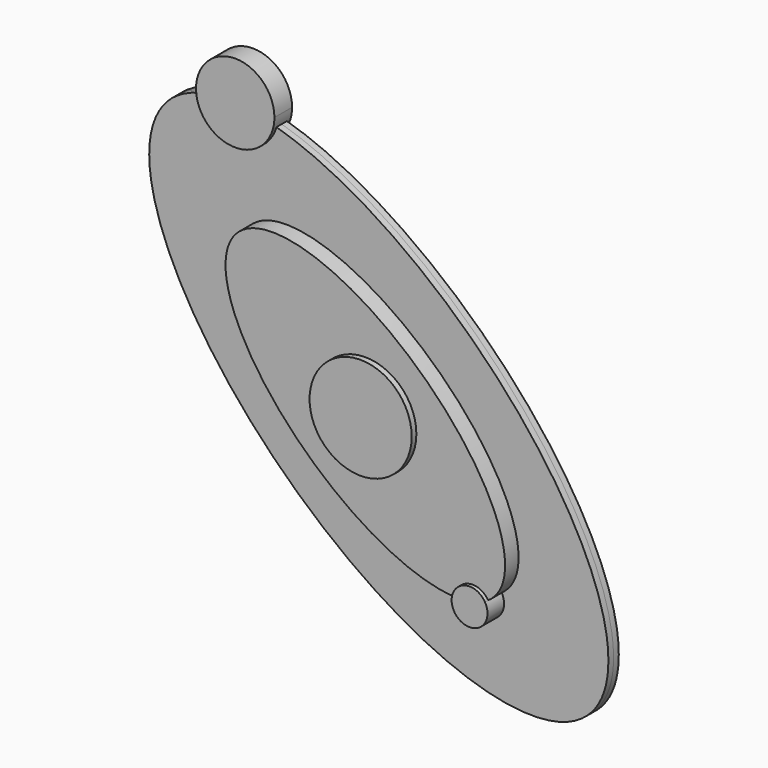
from build123d import *

# Parameters (mm, degrees)
F0_R     = 9.9911429725
F1_DEPTH = 4.572
F2_DEPTH = 1.27
F3_DEPTH = 2.159
F4_DEPTH = 5.334
F5_DEPTH = 5.715


with BuildPart() as f1:
    # F0 (on Front) → F1 (new body, symmetric)
    with BuildSketch(Plane.XZ):
        with BuildLine():
            add(Edge.make_bspline(
                [(24.0256715913, -24.0862835764), (37.8362153163, -14.8498020052), (11.6992033111, 10.0651317638), (-14.4378086941, 34.9800655329), (-25.3313519061, 22.9629725218)],
                knots=[3.0299304445, 3.0299304445, 3.0299304445, 4.6565578758, 4.6565578758, 6.2831853072, 6.2831853072, 6.2831853072], degree=2, weights=[1, 0.68709457, 1, 0.68709457, 1]))
            add(Edge.make_bspline(
                [(-25.3313519061, 22.9629725218), (-33.3755919456, 14.0890571319), (-16.1354711317, -5.4583110371), (1.1046496822, -25.0056792062), (17.5079205841, -25.6094847422)],
                knots=[0, 0, 0, 1.3259269599, 1.3259269599, 2.6518539199, 2.6518539199, 2.6518539199], degree=2, weights=[1, 0.7881718057, 1, 0.7881718057, 1]))
            ThreePointArc((17.5079205841, -25.6094847422), (20.2082141624, -22.4577219219), (24.0256715913, -24.0862835764))
        make_face()
        Circle(F0_R, mode=Mode.SUBTRACT)
    extrude(amount=F1_DEPTH, both=True)

    # F0 (on Front) → F2 (join, symmetric)
    with BuildSketch(Plane.XZ):
        with BuildLine():
            add(Edge.make_bspline(
                [(-34.973748483, 42.7912469007), (-38.9398495635, 41.8233210223), (-41.3951352239, 39.2327047884)],
                knots=[6.003713608, 6.003713608, 6.003713608, 6.2831853072, 6.2831853072, 6.2831853072], degree=2, weights=[1, 0.990252822, 1]))
            add(Edge.make_bspline(
                [(-41.3951352239, 39.2327047884), (-64.7472102278, 14.5935087972), (-5.026258058, -28.7696901063), (54.6946941118, -72.1328890099), (44.2403631424, -22.9469660632), (33.7860321731, 26.2389568835), (-20.0170077048, 41.7593431913)],
                knots=[0, 0, 0, 1.8577548126, 1.8577548126, 3.7155096253, 3.7155096253, 5.5732644379, 5.5732644379, 5.5732644379], degree=2, weights=[1, 0.5987334989, 1, 0.5987334989, 1, 0.5987334989, 1]))
            ThreePointArc((-20.0170077048, 41.7593431913), (-27.9123329766, 36.2318182758), (-34.973748483, 42.7912469007))
        make_face()
        with BuildLine():
            add(Edge.make_bspline(
                [(-25.3313519061, 22.9629725218), (-33.3755919456, 14.0890571319), (-16.1354711317, -5.4583110371), (1.1046496822, -25.0056792062), (17.5079205841, -25.6094847422)],
                knots=[0, 0, 0, 1.3259269599, 1.3259269599, 2.6518539199, 2.6518539199, 2.6518539199], degree=2, weights=[1, 0.7881718057, 1, 0.7881718057, 1]))
            add(Edge.make_bspline(
                [(24.0256715913, -24.0862835764), (37.8362153163, -14.8498020052), (11.6992033111, 10.0651317638), (-14.4378086941, 34.9800655329), (-25.3313519061, 22.9629725218)],
                knots=[3.0299304445, 3.0299304445, 3.0299304445, 4.6565578758, 4.6565578758, 6.2831853072, 6.2831853072, 6.2831853072], degree=2, weights=[1, 0.68709457, 1, 0.68709457, 1]))
            ThreePointArc((24.0256715913, -24.0862835764), (24.3908403493, -24.9474351534), (24.5155166316, -25.8744659432))
            ThreePointArc((24.5155166316, -25.8744659432), (20.8741233968, -29.3807680338), (17.5079205841, -25.6094847422))
        make_face(mode=Mode.SUBTRACT)
        with BuildLine():
            ThreePointArc((-34.973748483, 42.7912469007), (-27.9123329766, 36.2318182758), (-20.0170077048, 41.7593431913))
            add(Edge.make_bspline(
                [(-20.0170077048, 41.7593431913), (-28.8093975915, 44.2956550413), (-34.973748483, 42.7912469007)],
                knots=[5.5732644379, 5.5732644379, 5.5732644379, 6.003713608, 6.003713608, 6.003713608], degree=2, weights=[1, 0.9769284549, 1]))
        make_face()
    extrude(amount=F2_DEPTH, both=True)

    # F0 (on Front) → F3 (join, symmetric)
    with BuildSketch(Plane.XZ):
        with BuildLine():
            ThreePointArc((-34.973748483, 42.7912469007), (-27.9123329766, 36.2318182758), (-20.0170077048, 41.7593431913))
            add(Edge.make_bspline(
                [(-20.0170077048, 41.7593431913), (-28.8093975915, 44.2956550413), (-34.973748483, 42.7912469007)],
                knots=[5.5732644379, 5.5732644379, 5.5732644379, 6.003713608, 6.003713608, 6.003713608], degree=2, weights=[1, 0.9769284549, 1]))
        make_face()
        with BuildLine():
            add(Edge.make_bspline(
                [(-20.0170077048, 41.7593431913), (-28.8093975915, 44.2956550413), (-34.973748483, 42.7912469007)],
                knots=[5.5732644379, 5.5732644379, 5.5732644379, 6.003713608, 6.003713608, 6.003713608], degree=2, weights=[1, 0.9769284549, 1]))
            ThreePointArc((-20.0170077048, 41.7593431913), (-19.7929209788, 42.8094331248), (-19.7177338437, 43.880530984))
            ThreePointArc((-19.7177338437, 43.880530984), (-27.9306573409, 51.5279573891), (-34.973748483, 42.7912469007))
        make_face()
    extrude(amount=F3_DEPTH, both=True)

    # F0 (on Front) → F4 (join, symmetric)
    with BuildSketch(Plane.XZ):
        with BuildLine():
            add(Edge.make_bspline(
                [(17.5079205841, -25.6094847422), (21.5269517877, -25.7574255587), (24.0256715913, -24.0862835764)],
                knots=[2.6518539199, 2.6518539199, 2.6518539199, 3.0299304445, 3.0299304445, 3.0299304445], degree=2, weights=[1, 0.9821854137, 1]))
            ThreePointArc((17.5079205841, -25.6094847422), (20.8741233968, -29.3807680338), (24.5155166316, -25.8744659432))
            ThreePointArc((24.5155166316, -25.8744659432), (24.3908403493, -24.9474351534), (24.0256715913, -24.0862835764))
        make_face()
        with BuildLine():
            ThreePointArc((24.0256715913, -24.0862835764), (20.2082141624, -22.4577219219), (17.5079205841, -25.6094847422))
            add(Edge.make_bspline(
                [(17.5079205841, -25.6094847422), (21.5269517877, -25.7574255587), (24.0256715913, -24.0862835764)],
                knots=[2.6518539199, 2.6518539199, 2.6518539199, 3.0299304445, 3.0299304445, 3.0299304445], degree=2, weights=[1, 0.9821854137, 1]))
        make_face()
    extrude(amount=F4_DEPTH, both=True)

    # F0 (on Front) → F5 (join, symmetric)
    with BuildSketch(Plane.XZ):
        Circle(F0_R)
    extrude(amount=F5_DEPTH, both=True)


solid = f1.part
